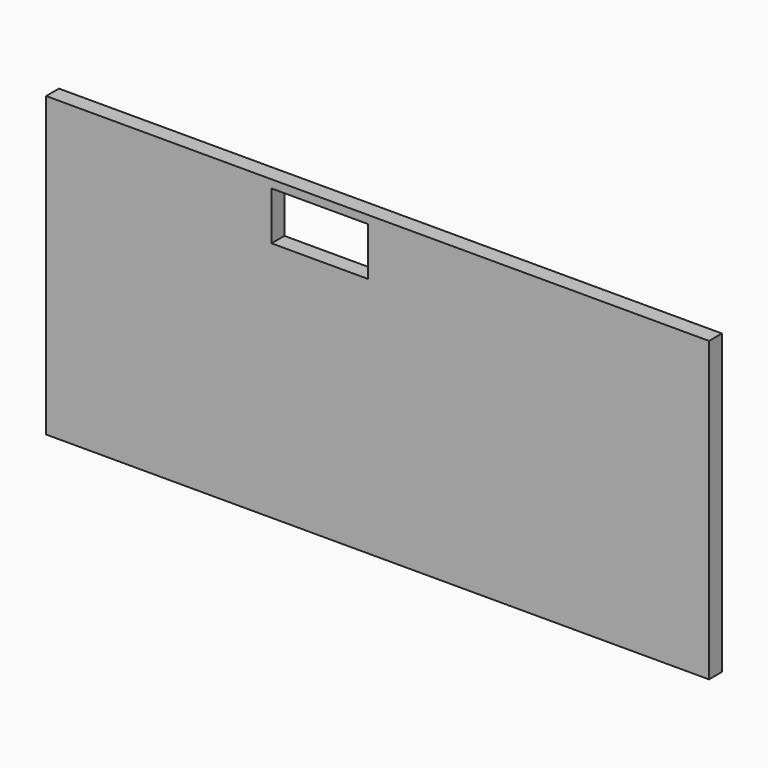
from build123d import *

# Parameters (mm, degrees)
F0_W      = 18288
F0_H      = 5486.4
F1_DEPTH  = 101.6
F2_W      = 4953
F2_H      = 152.4
F2_W_2    = 152.4
F2_H_2    = 3357.5625
F3_DEPTH  = 2426.49375
F4_DEPTH  = 152.4
F5_DEPTH  = 152.4
F6_W      = 4953
F6_H      = 152.4
F7_DEPTH  = 2350.29375
F8_DEPTH  = 76.2
F9_W      = 381
F9_H      = 279.4
F10_DEPTH = 2350.29375
F11_DEPTH = 101.6
F12_DEPTH = 101.6
F13_DEPTH = 275.43252
F14_DEPTH = 275.43252
F15_DEPTH = 25.4
F16_W     = 762
F16_H     = 254
F17_DEPTH = 2128.8385
F18_DEPTH = 190.5
F19_DEPTH = 63.5
F20_W     = 254
F20_H     = 304.8
F21_DEPTH = 152.401
F22_W     = 281.7354995728
F22_H     = 304.8
F23_DEPTH = 152.401
F24_DEPTH = 304.8
F25_DEPTH = 304.8
F26_DEPTH = 25.4
F27_DEPTH = 25.4
F28_DEPTH = 12.7
F29_DEPTH = 12.7
F30_W     = 127
F30_H     = 2350.29375
F31_DEPTH = 12907.16748
F32_W     = 1574.8
F32_H     = 2133.6
F33_DEPTH = 3230.5635
F34_DEPTH = 1320.8
F35_DEPTH = 1320.8
F36_DEPTH = 120.65
F37_DEPTH = 76.201
F38_DEPTH = 190.5
F39_DEPTH = 190.5
F40_DEPTH = 76.2
F41_DEPTH = 406.4
F42_DEPTH = 406.4
F43_DEPTH = 76.2
F44_DEPTH = 60.96
F45_DEPTH = 25.4
F46_DEPTH = 63.5
F47_DEPTH = 101.6
F48_DEPTH = 12907.16748
F49_DEPTH = 152.4
F51_DEPTH = 533.4


# Not quite as in the source:
# - a feature of the source that left no trace in its solid (it failed there, or was rolled back) is left out
# - a pattern or mirror of a feature is missing from the dataset's text; its kind, count and spacing are read off the source's solid


with BuildPart() as f1:
    # F0 (on Top) → F1 (new body)
    with BuildSketch(Plane.XY):
        with Locations((9144, 2743.2)):
            Rectangle(F0_W, F0_H)
    extrude(amount=F1_DEPTH)

    # F2 (on face) → F3 (join)
    with BuildSketch(Plane.XY.offset(101.6)):
        with Locations((15811.5, 2052.6375)):
            Rectangle(F2_W, F2_H)
        with Locations((13258.8, 3807.61875)):
            Rectangle(F2_W_2, F2_H_2)
        with Locations((13258.8, 2052.6375)):
            Rectangle(F2_W_2, F2_H)
    extrude(amount=F3_DEPTH)

    # F4 (add): a face of the model
    f4_faces = [f1.faces().sort_by_distance(p)[0] for p in [
        (18288, 60.4084786837, 50.8),
    ]]
    extrude(f4_faces, amount=F4_DEPTH)

    # F5 (add): a face of the model
    f5_faces = [f1.faces().sort_by_distance(p)[0] for p in [
        (15887.7, 5486.4, 82.9871117188),
    ]]
    extrude(f5_faces, amount=F5_DEPTH)

    # F6 (on face) → F7 (join)
    with BuildSketch(Plane.XY.offset(101.6)):
        with Locations((15811.5, 5562.6)):
            Rectangle(F6_W, F6_H)
        Polygon((18288, 2128.8375), (18440.4, 2128.8375), (18440.4, 5638.8), (18288, 5638.8), (18288, 5486.4), align=None)
    extrude(amount=F7_DEPTH)

    # F8 (cut): a face of the model
    f8_faces = [f1.faces().sort_by_distance(p)[0] for p in [
        (13270.9239827069, 3883.81875, 2528.09375),
    ]]
    extrude(f8_faces, amount=-F8_DEPTH, mode=Mode.SUBTRACT)

    # F9 (on face) → F10 (join, through all)
    with BuildSketch(Plane.XY.offset(101.6)):
        with Locations((18097.5, 5346.7)):
            Rectangle(F9_W, F9_H)
    extrude(amount=F10_DEPTH)

    # F11 (add): a face of the model
    f11_faces = [f1.faces().sort_by_distance(p)[0] for p in [
        (18097.5, 5207, 1276.746875),
    ]]
    extrude(f11_faces, amount=F11_DEPTH)

    # F12 (cut): a face of the model
    f12_faces = [f1.faces().sort_by_distance(p)[0] for p in [
        (17907, 5295.9, 1276.746875),
    ]]
    extrude(f12_faces, amount=-F12_DEPTH, mode=Mode.SUBTRACT)

    # F13 (add): a face of the model
    f13_faces = [f1.faces().sort_by_distance(p)[0] for p in [
        (13182.6, 3807.61875, 1276.746875),
    ]]
    extrude(f13_faces, amount=F13_DEPTH)

    # F14 (cut): a face of the model
    f14_faces = [f1.faces().sort_by_distance(p)[0] for p in [
        (13335, 3807.61875, 1276.746875),
    ]]
    extrude(f14_faces, amount=-F14_DEPTH, mode=Mode.SUBTRACT)

    # F15 (cut): a face of the model
    f15_faces = [f1.faces().sort_by_distance(p)[0] for p in [
        (15673.78374, 1976.4375, 1276.746875),
    ]]
    extrude(f15_faces, amount=-F15_DEPTH, mode=Mode.SUBTRACT)

    # F16 (on face) → F17 (cut, through all)
    with BuildSketch(Plane(origin=(0, 2128.8375, 0), x_dir=(-1, 0, 0), z_dir=(0, 1, 0))):
        with Locations((-14812.16748, 2070.89375)):
            Rectangle(F16_W, F16_H)
    extrude(amount=-F17_DEPTH, mode=Mode.SUBTRACT)

    # F18 (cut): a face of the model
    f18_faces = [f1.faces().sort_by_distance(p)[0] for p in [
        (14812.16748, 2065.3375, 2197.89375),
    ]]
    extrude(f18_faces, amount=-F18_DEPTH, mode=Mode.SUBTRACT)

    # F19 (add): a face of the model
    f19_faces = [f1.faces().sort_by_distance(p)[0] for p in [
        (14812.16748, 2065.3375, 1943.89375),
    ]]
    extrude(f19_faces, amount=F19_DEPTH)

    # F20 (on face) → F21 (cut, through all)
    with BuildSketch(Plane(origin=(18288, 0, 0), x_dir=(0, -1, 0), z_dir=(-1, 0, 0))):
        with Locations((-4978.4, 2223.29375)):
            Rectangle(F20_W, F20_H)
    extrude(amount=-F21_DEPTH, mode=Mode.SUBTRACT)

    # F22 (on face) → F23 (cut, through all)
    with BuildSketch(Plane(origin=(18288, 0, 0), x_dir=(0, -1, 0), z_dir=(-1, 0, 0))):
        with Locations((-3747.6677497864, 2223.29375)):
            Rectangle(F22_W, F22_H)
    extrude(amount=-F23_DEPTH, mode=Mode.SUBTRACT)

    # F24 (cut): a face of the model
    f24_faces = [f1.faces().sort_by_distance(p)[0] for p in [
        (18364.2, 3888.5354995728, 2223.29375),
    ]]
    extrude(f24_faces, amount=-F24_DEPTH, mode=Mode.SUBTRACT)

    # F25 (add): a face of the model
    f25_faces = [f1.faces().sort_by_distance(p)[0] for p in [
        (18364.2, 3606.8, 2223.29375),
    ]]
    extrude(f25_faces, amount=F25_DEPTH)

    # F26 (add): a face of the model
    f26_faces = [f1.faces().sort_by_distance(p)[0] for p in [
        (18364.2, 4193.3354995728, 2223.29375),
    ]]
    extrude(f26_faces, amount=F26_DEPTH)

    # F27 (cut): a face of the model
    f27_faces = [f1.faces().sort_by_distance(p)[0] for p in [
        (18364.2, 3911.6, 2223.29375),
    ]]
    extrude(f27_faces, amount=-F27_DEPTH, mode=Mode.SUBTRACT)

    # F28 (cut): a face of the model
    f28_faces = [f1.faces().sort_by_distance(p)[0] for p in [
        (18364.2, 3886.2, 2223.29375),
    ]]
    extrude(f28_faces, amount=-F28_DEPTH, mode=Mode.SUBTRACT)

    # F29 (add): a face of the model
    f29_faces = [f1.faces().sort_by_distance(p)[0] for p in [
        (18364.2, 4167.9354995728, 2223.29375),
    ]]
    extrude(f29_faces, amount=F29_DEPTH)

    # F30 (on face) → F31 (join, through all)
    with BuildSketch(Plane(origin=(12907.16748, 0, 0), x_dir=(0, -1, 0), z_dir=(-1, 0, 0))):
        with Locations((-2471.7375, 1276.746875)):
            Rectangle(F30_W, F30_H)
    extrude(amount=F31_DEPTH)

    # F32 (on face) → F33 (cut, through all)
    with BuildSketch(Plane.XZ.offset(-2408.2375)):
        with Locations((12018.16748, 1168.4)):
            Rectangle(F32_W, F32_H)
    extrude(amount=-F33_DEPTH, mode=Mode.SUBTRACT)

    # F34 (cut): a face of the model
    f34_faces = [f1.faces().sort_by_distance(p)[0] for p in [
        (11230.76748, 2471.7375, 1168.4),
    ]]
    extrude(f34_faces, amount=-F34_DEPTH, mode=Mode.SUBTRACT)

    # F35 (add): a face of the model
    f35_faces = [f1.faces().sort_by_distance(p)[0] for p in [
        (12805.56748, 2471.7375, 1168.4),
    ]]
    extrude(f35_faces, amount=F35_DEPTH)

    # F36 (add): a face of the model
    f36_faces = [f1.faces().sort_by_distance(p)[0] for p in [
        (18364.2, 4014.3677497864, 2070.89375),
    ]]
    extrude(f36_faces, amount=F36_DEPTH)

    # F37 (cut, through all): a face of the model
    f37_faces = [f1.faces().sort_by_distance(p)[0] for p in [
        (18364.2, 4014.3677497864, 2375.69375),
    ]]
    extrude(f37_faces, amount=-F37_DEPTH, mode=Mode.SUBTRACT)

    # F38 (cut): a face of the model
    f38_faces = [f1.faces().sort_by_distance(p)[0] for p in [
        (18364.2, 4978.4, 2070.89375),
    ]]
    extrude(f38_faces, amount=-F38_DEPTH, mode=Mode.SUBTRACT)

    # F39 (add): a face of the model
    f39_faces = [f1.faces().sort_by_distance(p)[0] for p in [
        (18364.2, 4978.4, 2375.69375),
    ]]
    extrude(f39_faces, amount=F39_DEPTH)

    # F40 (cut): a face of the model
    f40_faces = [f1.faces().sort_by_distance(p)[0] for p in [
        (18364.2, 4978.4, 2185.19375),
    ]]
    extrude(f40_faces, amount=-F40_DEPTH, mode=Mode.SUBTRACT)

    # F41 (cut): a face of the model
    f41_faces = [f1.faces().sort_by_distance(p)[0] for p in [
        (15193.16748, 2065.3375, 2197.89375),
    ]]
    extrude(f41_faces, amount=-F41_DEPTH, mode=Mode.SUBTRACT)

    # F42 (add): a face of the model
    f42_faces = [f1.faces().sort_by_distance(p)[0] for p in [
        (14431.16748, 2065.3375, 2197.89375),
    ]]
    extrude(f42_faces, amount=F42_DEPTH)

    # F43 (cut): a face of the model
    f43_faces = [f1.faces().sort_by_distance(p)[0] for p in [
        (18364.2, 3873.5, 2321.71875),
    ]]
    extrude(f43_faces, amount=-F43_DEPTH, mode=Mode.SUBTRACT)

    # F44 (cut): a face of the model
    f44_faces = [f1.faces().sort_by_distance(p)[0] for p in [
        (18364.2, 4155.2354995728, 2321.71875),
    ]]
    extrude(f44_faces, amount=-F44_DEPTH, mode=Mode.SUBTRACT)

    # F45 (add): a face of the model
    f45_faces = [f1.faces().sort_by_distance(p)[0] for p in [
        (18364.2, 4978.4, 1880.39375),
    ]]
    extrude(f45_faces, amount=F45_DEPTH)

    # F46 (cut): a face of the model
    f46_faces = [f1.faces().sort_by_distance(p)[0] for p in [
        (18364.2, 4978.4, 2261.39375),
    ]]
    extrude(f46_faces, amount=-F46_DEPTH, mode=Mode.SUBTRACT)

    # F47 (cut, through all): a face of the model
    f47_faces = [f1.faces().sort_by_distance(p)[0] for p in [
        (9220.2, 2819.4, 0),
    ]]
    extrude(f47_faces, amount=-F47_DEPTH, mode=Mode.SUBTRACT)

    # F48 (cut, through all): a face of the model
    f48_faces = [f1.faces().sort_by_distance(p)[0] for p in [
        (0, 2471.7375, 1276.746875),
    ]]
    extrude(f48_faces, amount=-F48_DEPTH, mode=Mode.SUBTRACT)

    # F49 (cut, through all): a face of the model
    f49_faces = [f1.faces().sort_by_distance(p)[0] for p in [
        (12907.16748, 3820.31875, 1276.746875),
    ]]
    f49 = extrude(f49_faces, amount=-F49_DEPTH, mode=Mode.SUBTRACT)

    # F49_copies: F49 across plane
    add(f49.mirror(Plane(origin=(15673.78374, 0, 0), x_dir=(0, 0, 1), z_dir=(1, 0, 0))), mode=Mode.SUBTRACT)

    # F51 (cut, through all): a face of the model
    f51_faces = [f1.faces().sort_by_distance(p)[0] for p in [
        (15673.78374, 5638.8, 1276.746875),
    ]]
    extrude(f51_faces, amount=-F51_DEPTH, mode=Mode.SUBTRACT)


solid = f1.part
